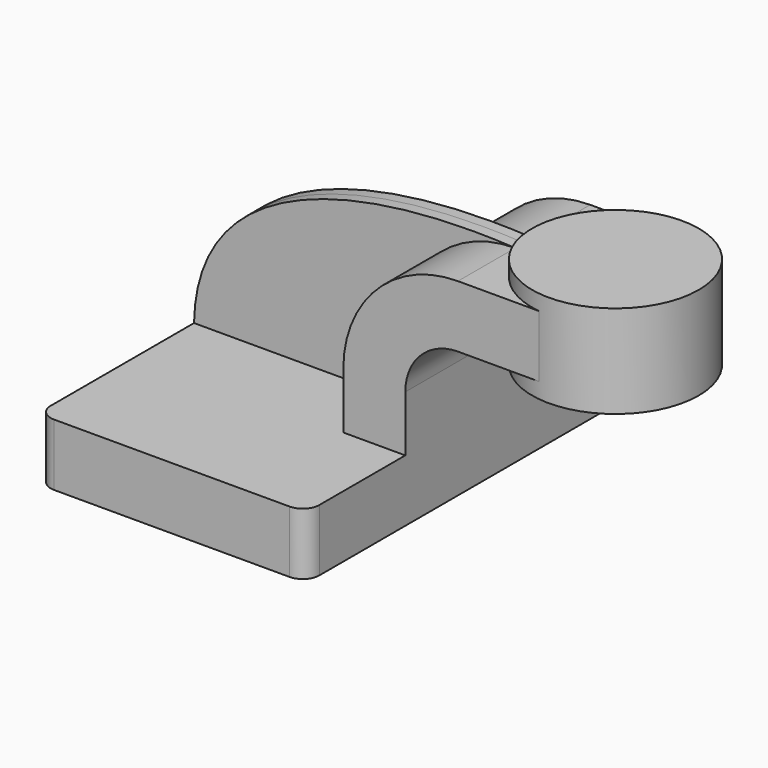
from build123d import *

# Parameters (mm, degrees)
F1_DEPTH = 63.5
F2_DEPTH = 25.4
F3_DEPTH = 3.3655
F0_W     = 25.2081867933
F0_H     = 19.05
F4_DEPTH = 25.4
F6_R     = 5.08


# Not quite as in the source:
# - a feature names something its author has since deleted; it is built from what else it names


with BuildPart() as f1:
    # F0 (on Front) → F1 (new body, symmetric)
    with BuildSketch(Plane.XZ):
        Polygon((-41.275, -9.525), (41.275, -9.525), (41.275, 9.525), (22.225, 9.525), (-41.275, 9.525), align=None)
    extrude(amount=F1_DEPTH, both=True)

    # F0 (on Front) → F2 (join, symmetric)
    with BuildSketch(Plane.XZ):
        with BuildLine():
            Line((22.225, 9.525), (41.275, 9.525))
            Line((41.275, 9.525), (41.275, 26.6985158606))
            ThreePointArc((41.275, 26.6985158606), (46.0130410873, 38.1371589127), (57.4516841394, 42.8752))
            Line((57.4516841394, 42.8752), (60.325, 42.8752))
            Line((60.325, 42.8752), (60.325, 61.9252))
            Line((60.325, 61.9252), (57.4516841394, 61.9252))
            ThreePointArc((57.4516841394, 61.9252), (32.5426569057, 51.6075430943), (22.225, 26.6985158606))
            Line((22.225, 26.6985158606), (22.225, 9.525))
        make_face()
    extrude(amount=F2_DEPTH, both=True)

    # F0 (on Front) → F3 (join, symmetric)
    with BuildSketch(Plane.XZ):
        with BuildLine():
            add(Edge.make_bspline(
                [(-41.275, 9.525), (-40.5068695545, 53.2762855291), (10.412055999, 64.5915940404), (57.4516841394, 61.9252)],
                knots=[0, 0, 0, 0, 111.7709225211, 111.7709225211, 111.7709225211, 111.7709225211], degree=3))
            Line((-41.275, 9.525), (22.225, 9.525))
            Line((22.225, 9.525), (22.225, 26.6985158606))
            ThreePointArc((22.225, 26.6985158606), (32.5426569057, 51.6075430943), (57.4516841394, 61.9252))
        make_face()
    extrude(amount=F3_DEPTH, both=True)

    # F0 (on Front) → F4 (join, symmetric)
    with BuildSketch(Plane.XZ):
        with Locations((72.9290933967, 52.4002)):
            Rectangle(F0_W, F0_H)
    extrude(amount=F4_DEPTH, both=True)

    # F0 (on Front) → F5 (revolve)
    with BuildSketch(Plane.XZ):
        Polygon((85.5331867933, 66.675), (85.5331867933, 61.9252), (85.5331867933, 42.8752), (85.5331867933, 38.1), (111.125, 38.1), (111.125, 66.675), align=None)
    revolve(axis=Axis((85.5331867933, 0, 52.3875), (0, 0, -1)))

    # F6
    f6_edges = [f1.edges().sort_by_distance(p)[0] for p in [
        (41.275, -63.5, 0),
        (-41.275, -63.5, 0),
        (41.275, 63.5, 0),
        (-41.275, 63.5, 0),
    ]]
    fillet(f6_edges, radius=F6_R)


solid = f1.part
